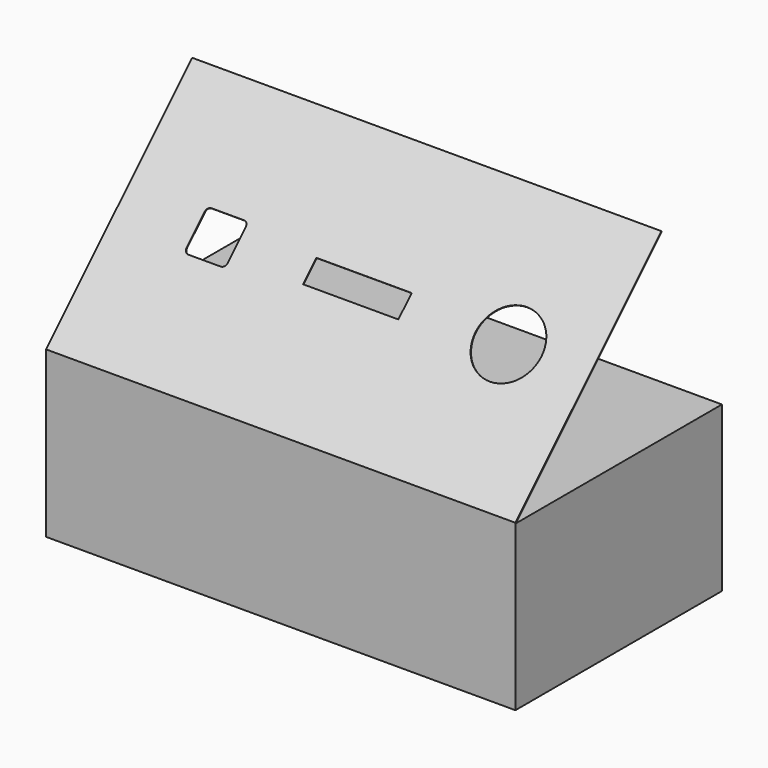
from build123d import *

# Parameters (mm, degrees)
F1_DEPTH = 127
F2_W     = 51.5939278
F2_H     = 12.7
F3_DEPTH = 0.4064


# Not quite as in the source:
# - the dataset's text gives a spline's control points without its knots; the knots are read off the source's solid


with BuildPart() as f1:
    # F0 (on Right) → F1 (new body, symmetric)
    with BuildSketch(Plane.YZ):
        Polygon((-139.7, 0), (0, 0), (0, 88.9), (-139.2936, 88.9), (-139.2936, 89.154), (-40.6298144724, 187.8177855276), (-40.9171826682, 188.1051537235), (-139.7, 89.3223363917), align=None)
    extrude(amount=F1_DEPTH, both=True)

    # F2 (on face) → F3 (cut, through all)
    with BuildSketch(Plane(origin=(0, -114.5111681959, 114.5111681959), x_dir=(1, 0, 0), z_dir=(0, -0.7071067812, 0.7071067812))):
        with BuildLine():
            add(Edge.make_bspline(
                [(-64.5206424843, 24.6188538049), (-64.0800032843, 25.0598232049), (-63.8233616843, 25.6795832049), (-63.8233616843, 26.3027976049)],
                knots=[1, 1, 1, 1, 2, 2, 2, 2], degree=3))
            Line((-63.8233616843, 26.3027976049), (-63.8233616843, 43.7652976049))
            add(Edge.make_bspline(
                [(-63.8233616843, 43.7652976049), (-63.8233616843, 44.3888676049), (-64.0800032843, 45.0082974049), (-64.5206424843, 45.4492668049)],
                knots=[0, 0, 0, 0, 1, 1, 1, 1], degree=3))
            add(Edge.make_bspline(
                [(-64.5206424843, 45.4492668049), (-64.9616118843, 45.8899060049), (-65.5806860843, 46.1465476049), (-66.2046116843, 46.1465476049)],
                knots=[1, 1, 1, 1, 2, 2, 2, 2], degree=3))
            Line((-66.2046116843, 46.1465476049), (-83.6671116843, 46.1465476049))
            add(Edge.make_bspline(
                [(-83.6671116843, 46.1465476049), (-84.2903260843, 46.1465476049), (-84.9097304843, 45.8899060049), (-85.3503696843, 45.4492668049), (-85.7913390843, 45.0082974049), (-86.0483616843, 44.3888676049), (-86.0483616843, 43.7652976049)],
                knots=[0, 0, 0, 0, 1, 1, 1, 2, 2, 2, 2], degree=3))
            Line((-86.0483616843, 43.7652976049), (-86.0483616843, 26.3027976049))
            add(Edge.make_bspline(
                [(-86.0483616843, 26.3027976049), (-86.0483616843, 25.6795832049), (-85.7913390843, 25.0598232049), (-85.3503696843, 24.6188538049)],
                knots=[0, 0, 0, 0, 1, 1, 1, 1], degree=3))
            add(Edge.make_bspline(
                [(-85.3503696843, 24.6188538049), (-84.9097304843, 24.1785448049), (-84.2903260843, 23.9215476049), (-83.6671116843, 23.9215476049)],
                knots=[1, 1, 1, 1, 2, 2, 2, 2], degree=3))
            Line((-83.6671116843, 23.9215476049), (-66.2046116843, 23.9215476049))
            add(Edge.make_bspline(
                [(-66.2046116843, 23.9215476049), (-65.5806860843, 23.9215476049), (-64.9616118843, 24.1785448049), (-64.5206424843, 24.6188538049)],
                knots=[0, 0, 0, 0, 1, 1, 1, 1], degree=3))
        make_face()
        with Locations((1.2642272157, 35.4309226049)):
            Rectangle(F2_W, F2_H)
        with BuildLine():
            add(Edge.make_bspline(
                [(95.6440867157, 48.0854566049), (92.3381497157, 51.3917238049), (87.6914483157, 53.3164596049), (83.0157655157, 53.3164596049)],
                knots=[7, 7, 7, 7, 8, 8, 8, 8], degree=3))
            add(Edge.make_bspline(
                [(83.0157655157, 53.3164596049), (78.3400827157, 53.3164596049), (73.6933305157, 51.3917238049), (70.3874189157, 48.0854566049)],
                knots=[0, 0, 0, 0, 1, 1, 1, 1], degree=3))
            add(Edge.make_bspline(
                [(70.3874189157, 48.0854566049), (67.0814819157, 44.7795196049), (65.1563905157, 40.1324626049), (65.1563905157, 35.4570846049), (65.1563905157, 30.7814018049), (67.0814819157, 26.1347004049), (70.3874189157, 22.8280776049)],
                knots=[1, 1, 1, 1, 2, 2, 2, 3, 3, 3, 3], degree=3))
            add(Edge.make_bspline(
                [(70.3874189157, 22.8280776049), (73.6933305157, 19.5221660049), (78.3400827157, 17.5977096049), (83.0157655157, 17.5977096049), (87.6914483157, 17.5977096049), (92.3381497157, 19.5221660049), (95.6440867157, 22.8280776049)],
                knots=[3, 3, 3, 3, 4, 4, 4, 5, 5, 5, 5], degree=3))
            add(Edge.make_bspline(
                [(95.6440867157, 22.8280776049), (98.9506841157, 26.1347004049), (100.8751405157, 30.7814018049), (100.8751405157, 35.4570846049), (100.8751405157, 40.1324626049), (98.9506841157, 44.7795196049), (95.6440867157, 48.0854566049)],
                knots=[5, 5, 5, 5, 6, 6, 6, 7, 7, 7, 7], degree=3))
        make_face()
    extrude(amount=-F3_DEPTH, mode=Mode.SUBTRACT)


solid = f1.part
